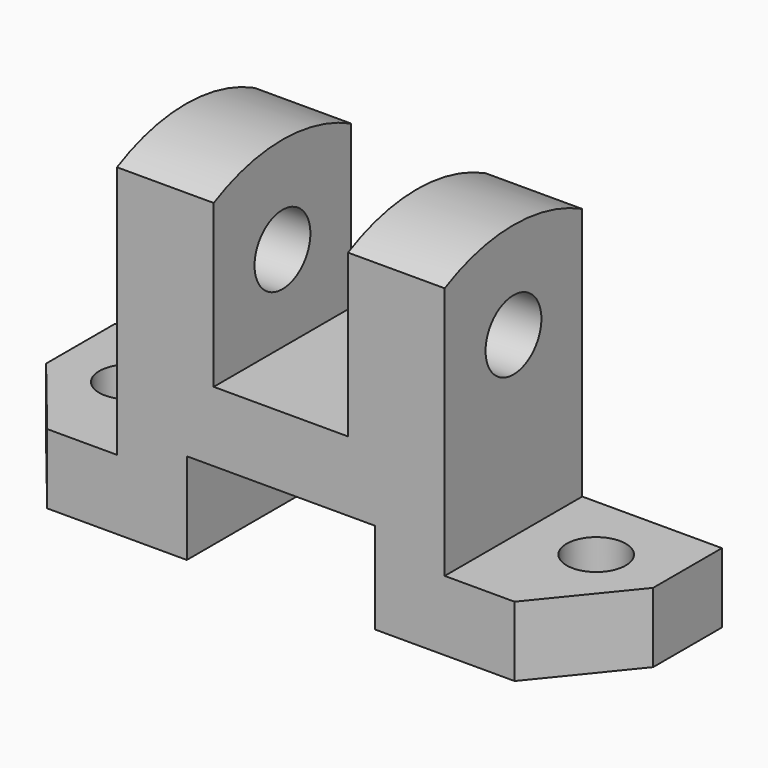
from build123d import *

# Parameters (mm, degrees)
F0_W      = 32
F0_H      = 13
F1_DEPTH  = 113
F2_W      = 35
F2_H      = 32
F3_DEPTH  = 17
F4_W      = 25
F4_H      = 30.1287648325
F4_H_2    = 18.8096150512
F4_W_2    = 26
F4_H_3    = 47.1287648325
F5_DEPTH  = 32.001
F6_R      = 5.5
F7_DEPTH  = 13.001
F8_R      = 5.5
F9_DEPTH  = 13.001
F10_R     = 6.5
F11_DEPTH = 87.001


with BuildPart() as f1:
    # F0 (on Right) → F1 (new body)
    with BuildSketch(Plane.YZ):
        with Locations((16, 6.5)):
            Rectangle(F0_W, F0_H)
        with BuildLine():
            Line((0, 60.1287648325), (0, 13))
            Line((0, 13), (32, 13))
            Line((32, 13), (32, 60.1287648325))
            ThreePointArc((32, 60.1287648325), (16, 64), (0, 60.1287648325))
        make_face()
    extrude(amount=F1_DEPTH)

    # F2 (on face) → F3 (cut)
    with BuildSketch(Plane(origin=(0, 0, 0), x_dir=(1, 0, 0), z_dir=(0, 0, -1))):
        with Locations((56.5, -16)):
            Rectangle(F2_W, F2_H)
    extrude(amount=-F3_DEPTH, mode=Mode.SUBTRACT)

    # F4 (on face) → F5 (cut, through all)
    with BuildSketch(Plane.XZ):
        with Locations((56.5, 45.0643824163)):
            Rectangle(F4_W, F4_H)
        with Locations((56.5, 69.5335723582)):
            Rectangle(F4_W, F4_H_2)
        with Locations((100, 36.5643824163)):
            Rectangle(F4_W_2, F4_H_3)
        with Locations((100, 69.5335723582)):
            Rectangle(F4_W_2, F4_H_2)
        with Locations((13, 69.5335723582)):
            Rectangle(F4_W_2, F4_H_2)
        with Locations((13, 36.5643824163)):
            Rectangle(F4_W_2, F4_H_3)
    extrude(amount=-F5_DEPTH, mode=Mode.SUBTRACT)

    # F6 (on face) → F7 (cut, through all)
    with BuildSketch(Plane.XY.offset(13)):
        Polygon((113, 0), (113, 16), (100, 0), align=None)
        with Locations((100, 19)):
            Circle(F6_R)
    extrude(amount=-F7_DEPTH, mode=Mode.SUBTRACT)

    # F8 (on face) → F9 (cut, through all)
    with BuildSketch(Plane.XY.offset(13)):
        with Locations((13, 19)):
            Circle(F8_R)
        Polygon((0, 16), (0, 0), (13, 0), align=None)
    extrude(amount=-F9_DEPTH, mode=Mode.SUBTRACT)

    # F10 (on face) → F11 (cut, through all)
    with BuildSketch(Plane.YZ.offset(87)):
        with Locations((16, 46)):
            Circle(F10_R)
    extrude(amount=-F11_DEPTH, mode=Mode.SUBTRACT)


solid = f1.part
